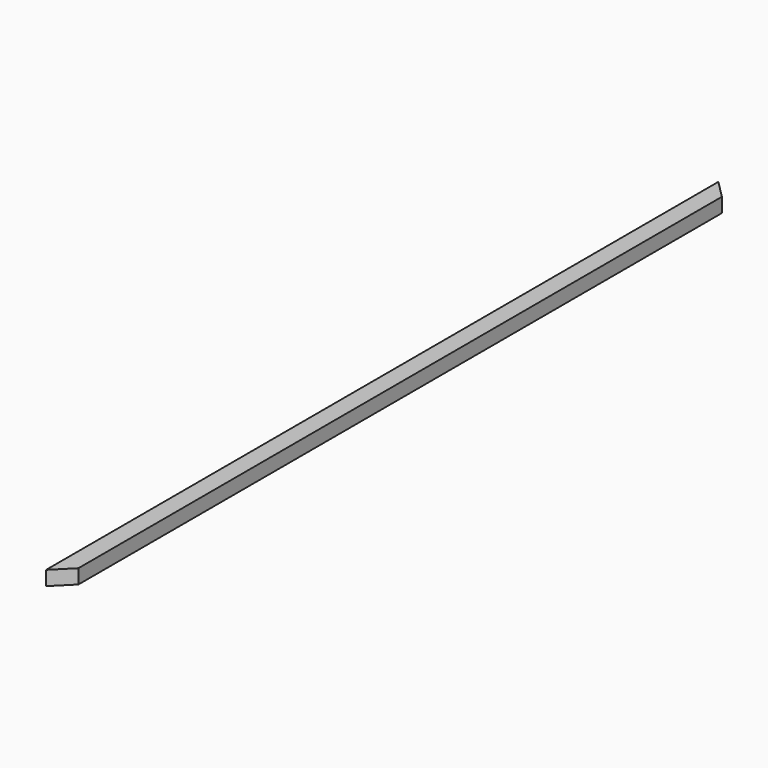
from build123d import *

# Parameters (mm, degrees)
F0_W     = 50
F0_H     = 40
F1_DEPTH = 2340
F2_SIZE2 = 49.99999
F2_SIZE  = 49.99999


# Not quite as in the source:
# - a fillet or chamfer is up to 0.001 mm smaller than in the source, because OpenCascade refuses the exact size


with BuildPart() as f1:
    # F0 (on Front) → F1 (new body)
    with BuildSketch(Plane.XZ):
        with Locations((25, 20)):
            Rectangle(F0_W, F0_H)
    extrude(amount=F1_DEPTH)

    # F2 (size 50 and 50 in the source; OpenCascade refuses exactly that, so slightly less here)
    f2_edges = [f1.edges().sort_by_distance(p)[0] for p in [
        (50, 0, 20),
        (50, -2340, 20),
    ]]
    chamfer(f2_edges, length=F2_SIZE, length2=F2_SIZE2)


solid = f1.part
